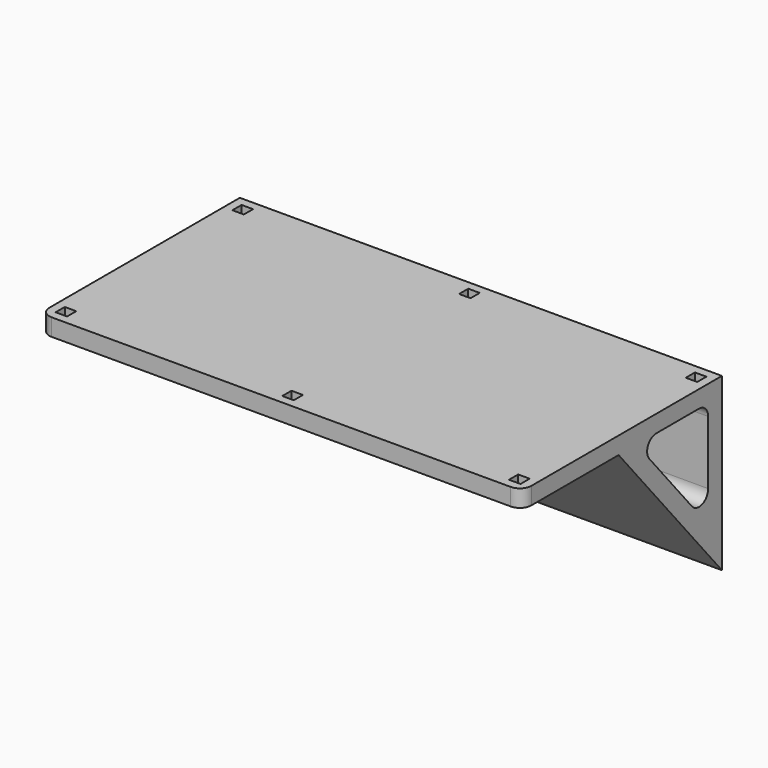
from build123d import *

# Parameters (mm, degrees)
F1_DEPTH = 84
F2_R     = 2
F3_R     = 2
F4_W     = 2
F4_H     = 2
F5_DEPTH = 4


# Not quite as in the source:
# - a feature names something its author has since deleted; it is built from what else it names


with BuildPart() as f1:
    # F0 (on Right) → F1 (new body)
    with BuildSketch(Plane.YZ):
        Polygon((0, 3), (0, 0), (21, 0), (43.497566339, -26.8115555092), (43.497566339, 3), (21, 3), align=None)
        Polygon((40.497566339, -18.5691232508), (24.916221868, 0), (40.497566339, 0), align=None, mode=Mode.SUBTRACT)
    extrude(amount=-F1_DEPTH)

    # F2
    f2_edges = [f1.edges().sort_by_distance(p)[0] for p in [
        (0, 0, 1.5),
        (-84, 0, 1.5),
    ]]
    fillet(f2_edges, radius=F2_R)

    # F3
    f3_edges = [f1.edges().sort_by_distance(p)[0] for p in [
        (-42, 40.497566, 0),
        (-42, 40.497566, -18.569123),
        (-42, 24.916222, 0),
    ]]
    fillet(f3_edges, radius=F3_R)

    # F4 (on face) → F5 (cut)
    with BuildSketch(Plane.XY.offset(3)):
        with Locations((-42, 40.997566339)):
            Rectangle(F4_W, F4_H)
        with Locations((-2.5, 40.997566339)):
            Rectangle(F4_W, F4_H)
        with Locations((-2.5, 2.5)):
            Rectangle(F4_W, F4_H)
        with Locations((-42, 2.4999999997)):
            Rectangle(F4_W, F4_H)
        with Locations((-81.5, 2.5)):
            Rectangle(F4_W, F4_H)
        with Locations((-81.5, 40.997566339)):
            Rectangle(F4_W, F4_H)
    extrude(amount=-F5_DEPTH, mode=Mode.SUBTRACT)


solid = f1.part
